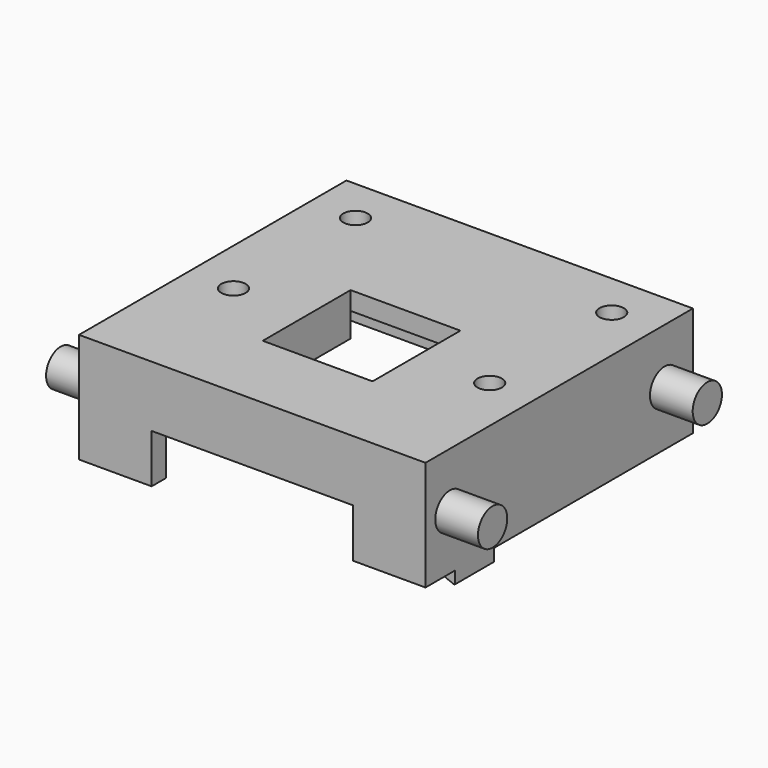
from build123d import *

# Parameters (mm, degrees)
F1_DEPTH    = 1.5
F2_DEPTH    = 9
F0_W        = 4.5
F0_H        = 4.5
F0_R        = 1
F3_DEPTH    = 3.5
F0_W_2      = 16.5
F0_H_2      = 1.5
F4_DEPTH    = 5
F5_R        = 1.5
F6_DEPTH    = 3.5
F8_R        = 3
F9_W        = 0.6
F9_H        = 4
F9_W_2      = 1.5
F9_W_3      = 4
F9_H_2      = 0.6
F9_H_3      = 1.5
F10_DEPTH   = 1
F11_SIZE2   = 2
F11_SIZE    = 0.8
F11_2_SIZE2 = 2
F11_2_SIZE  = 0.8
F12_SIZE2   = 0.8
F12_SIZE    = 2


# Not quite as in the source:
# - a feature names something its author has since deleted; it is built from what else it names


with BuildPart() as f1:
    # F0 (on Top) → F1 (new body)
    with BuildSketch(Plane.XY):
        Polygon((8.2, 12.2), (-8.2, 12.2), (-8.2, 7.7), (-12.7, 7.7), (-12.7, -0.25), (-8.2, -0.25), (-8.2, -4.75), (-12.7, -4.75), (-12.7, -12.2), (-8.25, -12.2), (8.25, -12.2), (12.7, -12.2), (12.7, -4.75), (8.2, -4.75), (8.2, -0.25), (12.7, -0.25), (12.7, 7.7), (8.2, 7.7), align=None)
        Polygon((-6.5, 2), (-4.5, 2), (4.5, 2), (6.5, 2), (6.5, -9), (-6.5, -9), align=None, mode=Mode.SUBTRACT)
    extrude(amount=-F1_DEPTH)



with BuildPart() as f2:
    # F0 (on Top) → F2 (new body)
    with BuildSketch(Plane.XY):
        Polygon((-12.7, 7.7), (-12.7, 12.2), (-8.2, 12.2), (8.2, 12.2), (12.7, 12.2), (12.7, 7.7), (12.7, -0.25), (12.7, -4.75), (12.7, -12.2), (8.25, -12.2), (8.25, -13.7), (14.2, -13.7), (14.2, 13.7), (-14.2, 13.7), (-14.2, -13.7), (-8.25, -13.7), (-8.25, -12.2), (-12.7, -12.2), (-12.7, -4.75), (-12.7, -0.25), align=None)
    extrude(amount=-F2_DEPTH)


with BuildPart() as f3:
    # F0 (on Top) → F3 (new body)
    with BuildSketch(Plane.XY):
        with Locations((10.45, 9.95)):
            Rectangle(F0_W, F0_H)
        with Locations((10.5, 10)):
            Circle(F0_R, mode=Mode.SUBTRACT)
    extrude(amount=-F3_DEPTH)


with BuildPart() as f3b:
    # F0 (on Top) → F3, piece 2 (new body)
    with BuildSketch(Plane.XY):
        with Locations((10.45, -2.5)):
            Rectangle(F0_W, F0_H)
        with Locations((10.5, -2.5)):
            Circle(F0_R, mode=Mode.SUBTRACT)
    extrude(amount=-F3_DEPTH)


with BuildPart() as f3c:
    # F0 (on Top) → F3, piece 3 (new body)
    with BuildSketch(Plane.XY):
        Polygon((-4.5, -7), (-4.5, 2), (-6.5, 2), (-6.5, -9), (6.5, -9), (6.5, 2), (4.5, 2), (4.5, -7), align=None)
    extrude(amount=-F3_DEPTH)


with BuildPart() as f3d:
    # F0 (on Top) → F3, piece 4 (new body)
    with BuildSketch(Plane.XY):
        with Locations((-10.45, 9.95)):
            Rectangle(F0_W, F0_H)
        with Locations((-10.5, 10)):
            Circle(F0_R, mode=Mode.SUBTRACT)
    extrude(amount=-F3_DEPTH)


with BuildPart() as f3e:
    # F0 (on Top) → F3, piece 5 (new body)
    with BuildSketch(Plane.XY):
        with Locations((-10.45, -2.5)):
            Rectangle(F0_W, F0_H)
        with Locations((-10.5, -2.5)):
            Circle(F0_R, mode=Mode.SUBTRACT)
    extrude(amount=-F3_DEPTH)


with BuildPart() as f1_1:
    add(f1.part)

    add(f2.part)  # F4 merges F2
    # F0 (on Top) → F4 (join)
    with BuildSketch(Plane.XY):
        with Locations((0, -12.95)):
            Rectangle(F0_W_2, F0_H_2)
    extrude(amount=-F4_DEPTH)

    # F5 (on face) → F6 (join)
    with BuildSketch(Plane(origin=(-14.2, 0, 0), x_dir=(0, -1, 0), z_dir=(-1, 0, 0))):
        with Locations((11.2, -4.5)):
            Circle(F5_R)
        with Locations((-10.8, -4.5)):
            Circle(F5_R)
    extrude(amount=F6_DEPTH)



with BuildPart() as f1_2:
    add(f1_1.part)

    add(f3.part)  # F7 merges F3

    add(f3b.part)  # F7 merges F3b

    add(f3c.part)  # F7 merges F3c

    add(f3d.part)  # F7 merges F3d

    add(f3e.part)  # F7 merges F3e
    # F7: F1 across plane
    add(f1_1.part.mirror(Plane.YZ))

    # F8
    f8_edges = [f1_2.edges().sort_by_distance(p)[0] for p in [
        (8.2, 7.7, -2.5),
        (-8.2, 7.7, -2.5),
    ]]
    fillet(f8_edges, radius=F8_R)

    # F9 (on face) → F10 (join)
    with BuildSketch(Plane(origin=(0, 0, -9), x_dir=(1, 0, 0), z_dir=(0, 0, -1))):
        with Locations((-12.4, 8.7)):
            Rectangle(F9_W, F9_H)
        with Locations((-13.45, 8.7)):
            Rectangle(F9_W_2, F9_H)
        with Locations((12.4, 8.7)):
            Rectangle(F9_W, F9_H)
        with Locations((13.45, 8.7)):
            Rectangle(F9_W_2, F9_H)
        with Locations((0, -11.9)):
            Rectangle(F9_W_3, F9_H_2)
        with Locations((0, -12.95)):
            Rectangle(F9_W_3, F9_H_3)
    extrude(amount=F10_DEPTH)

    # F11
    f11_edges = [f1_2.edges().sort_by_distance(p)[0] for p in [
        (-12.1, -8.7, -10),
    ]]
    f11_side = f1_2.faces().sort_by_distance((-12.1, -8.7, -9.5))[0]
    chamfer(f11_edges, length=F11_SIZE, length2=F11_SIZE2, reference=f11_side)

    # F11#2
    f11_2_edges = [f1_2.edges().sort_by_distance(p)[0] for p in [
        (0, 11.6, -10),
    ]]
    f11_2_side = f1_2.faces().sort_by_distance((0, 11.6, -9.5))[0]
    chamfer(f11_2_edges, length=F11_2_SIZE, length2=F11_2_SIZE2, reference=f11_2_side)

    # F12
    f12_edges = [f1_2.edges().sort_by_distance(p)[0] for p in [
        (12.1, -8.7, -10),
    ]]
    f12_side = f1_2.faces().sort_by_distance((13.15, -8.7, -10))[0]
    chamfer(f12_edges, length=F12_SIZE, length2=F12_SIZE2, reference=f12_side)


solid = f1_2.part
